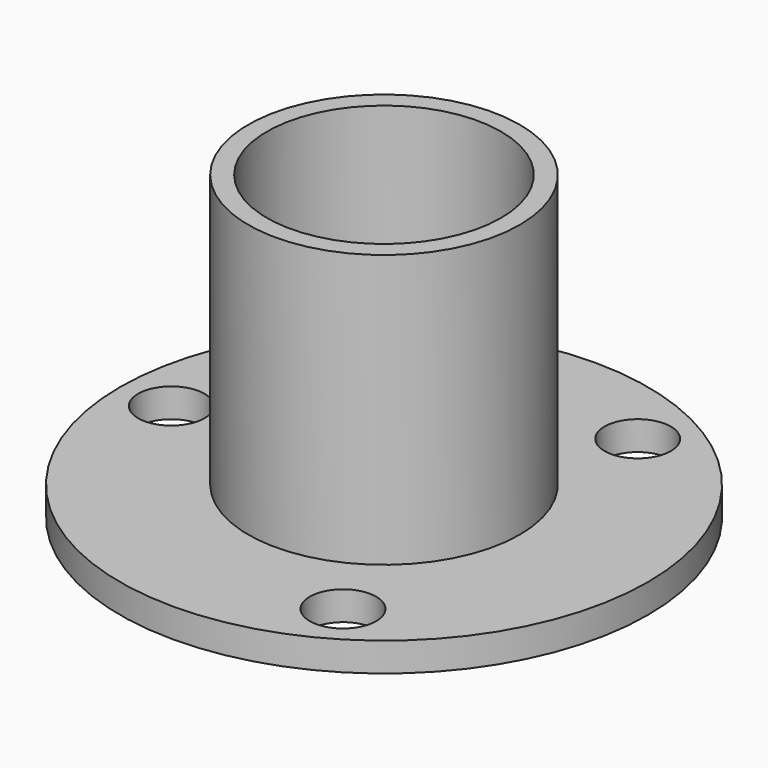
from build123d import *

# Parameters (mm, degrees)
F0_R            = 21.875
F0_R_2          = 11.25
F0_R_3          = 9.7
F1_DEPTH        = 2.4
F2_DEPTH        = 25
F3_D            = 5.5
F3_COPIES_COUNT = 3


# Not quite as in the source:
# - a pattern or mirror of a feature is missing from the dataset's text; its kind, count and spacing are read off the source's solid


with BuildPart() as f1:
    # F0 (on Top) → F1 (new body)
    with BuildSketch(Plane.XY):
        Circle(F0_R)
        Circle(F0_R_2, mode=Mode.SUBTRACT)
        Circle(F0_R_2)
        Circle(F0_R_3, mode=Mode.SUBTRACT)
    extrude(amount=F1_DEPTH)

    # F0 (on Top) → F2 (join)
    with BuildSketch(Plane.XY):
        Circle(F0_R_2)
        Circle(F0_R_3, mode=Mode.SUBTRACT)
    extrude(amount=F2_DEPTH)

    # F3 (through all)
    with Locations(Plane(origin=(0, 0, 0), x_dir=(1, 0, 0), z_dir=(0, 0, -1))):
        with Locations((-17.625, 0)):
            f3 = Hole(F3_D / 2)

    # F3_copies: F3 ×3 about axis
    f3_copies_axis = Axis((0, 0, 0), (0, 0, 1))
    for i in range(1, F3_COPIES_COUNT):
        add(f3.rotate(f3_copies_axis, i * 360 / F3_COPIES_COUNT), mode=Mode.SUBTRACT)


solid = f1.part
